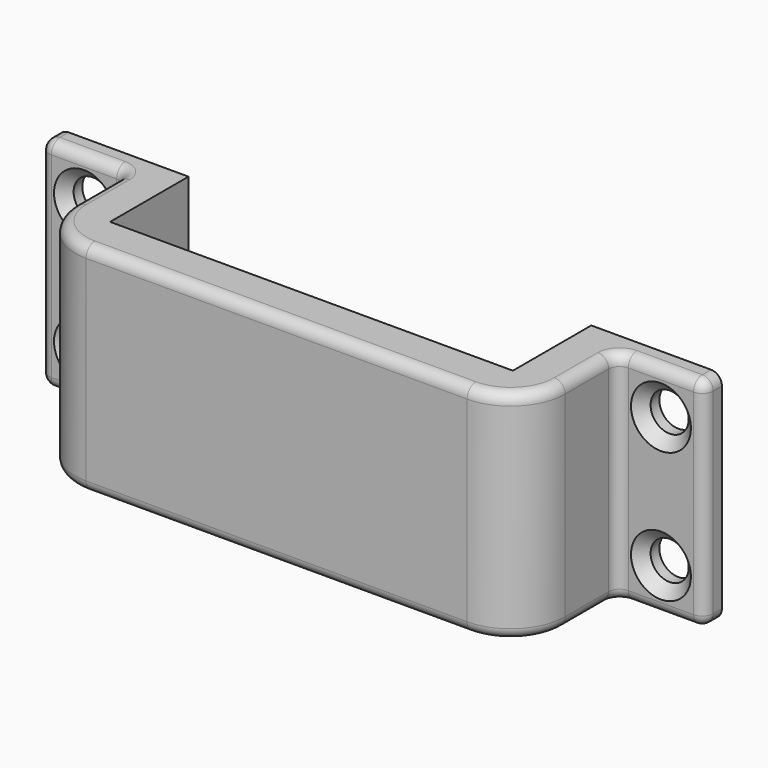
from build123d import *

# Parameters (mm, degrees)
F0_W           = 4
F0_H           = 20
F0_W_2         = 37
F1_DEPTH       = 4
F2_DEPTH       = 9
F3_W           = 8
F3_H           = 20
F4_DEPTH       = 2
F6_D           = 3.5
F6_CSINK_D     = 5.5
F6_CSINK_ANGLE = 90
F7_R           = 5
F8_R           = 1


with BuildPart() as f1:
    # F0 (on Front) → F1 (new body)
    with BuildSketch(Plane.XZ):
        with Locations((-20.5, 0)):
            Rectangle(F0_W, F0_H)
        Rectangle(F0_W_2, F0_H)
        with Locations((20.5, 0)):
            Rectangle(F0_W, F0_H)
    extrude(amount=F1_DEPTH)

    # F0 (on Front) → F2 (join)
    with BuildSketch(Plane.XZ):
        with Locations((-20.5, 0)):
            Rectangle(F0_W, F0_H)
        with Locations((20.5, 0)):
            Rectangle(F0_W, F0_H)
    extrude(amount=-F2_DEPTH)

    # F3 (on face) → F4 (join)
    with BuildSketch(Plane(origin=(0, 9, 0), x_dir=(-1, 0, 0), z_dir=(0, 1, 0))):
        with Locations((-26.5, 0)):
            Rectangle(F3_W, F3_H)
        with Locations((26.5, 0)):
            Rectangle(F3_W, F3_H)
    extrude(amount=-F4_DEPTH)

    # F6 (through all)
    with Locations(Plane.XZ.offset(-7)):
        with Locations((-26.5, -6), (-26.5, 6), (26.5, -6), (26.5, 6)):
            CounterSinkHole(F6_D / 2, F6_CSINK_D / 2, counter_sink_angle=F6_CSINK_ANGLE)

    # F7
    f7_edges = [f1.edges().sort_by_distance(p)[0] for p in [
        (22.5, -4, 0),
        (-22.5, -4, 0),
    ]]
    fillet(f7_edges, radius=F7_R)

    # F8
    f8_edges = [f1.edges().sort_by_distance(p)[0] for p in [
        (22.5, 7, 0),
        (-22.5, 7, 0),
        (26.5, 7, 10),
        (26.5, 7, -10),
        (30.5, 7, 0),
        (-30.5, 7, 0),
        (30.5, 8, 10),
        (30.5, 8, -10),
        (-30.5, 8, 10),
        (-30.5, 8, -10),
        (-22.5, 4, -10),
        (-21.035534, -2.535534, -10),
        (-26.5, 7, -10),
        (0, -4, -10),
        (21.035534, -2.535534, -10),
        (22.5, 4, -10),
        (-22.5, 4, 10),
        (-21.035534, -2.535534, 10),
        (-26.5, 7, 10),
        (0, -4, 10),
        (21.035534, -2.535534, 10),
        (22.5, 4, 10),
    ]]
    fillet(f8_edges, radius=F8_R)


solid = f1.part
